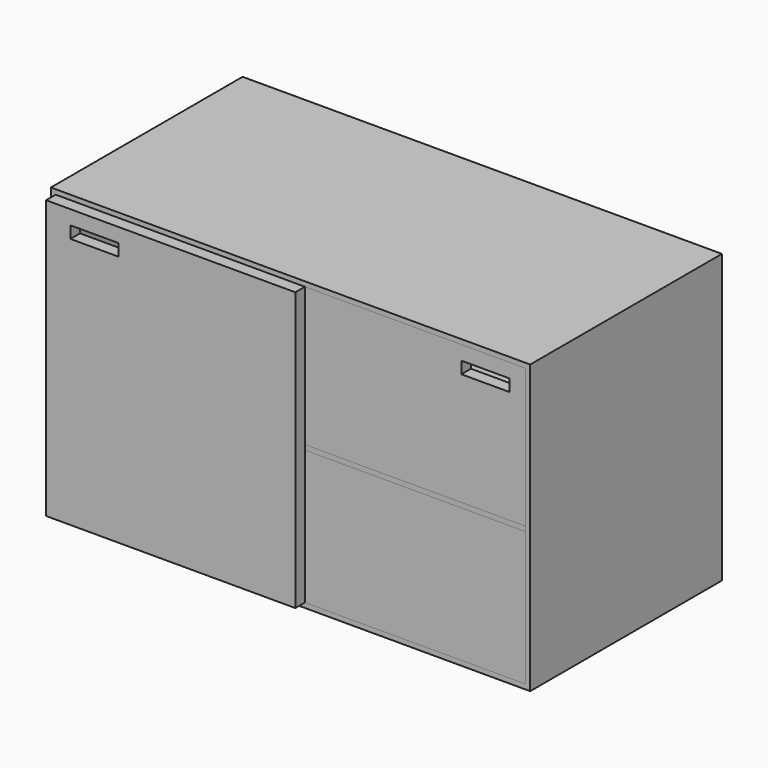
from build123d import *

# Parameters (mm, degrees)
F0_W          = 1000
F0_H          = 600
F1_DEPTH      = 500
F2_T          = -10
F3_W          = 460
F3_H          = 580
F3_W_2        = 60
F4_DEPTH      = 25
F5_DEPTH      = 25
F6_W          = 100
F6_H          = 25
F7_DEPTH      = 525.001
F7_DEPTH_BACK = 1899
F8_W          = 980
F8_H          = 10
F9_DEPTH      = 490
F10_W         = 10
F10_H         = 580
F11_DEPTH     = 490


# Not quite as in the source:
# - an extrude ends at something that could not be found from the text; its depth is read off the source's solid


with BuildPart() as f1:
    # F0 (on Front) → F1 (new body)
    with BuildSketch(Plane.XZ):
        with Locations((500, 300)):
            Rectangle(F0_W, F0_H)
    extrude(amount=F1_DEPTH)

    # F2
    f2_openings = [f1.faces().sort_by_distance(p)[0] for p in [
        (500, -500, 300),
    ]]
    offset(amount=F2_T, openings=f2_openings)


with BuildPart() as f4:
    # F3 (on face) → F4 (new body)
    with BuildSketch(Plane.XZ.offset(500)):
        with Locations((240, 300)):
            Rectangle(F3_W, F3_H)
        with Locations((500, 300)):
            Rectangle(F3_W_2, F3_H)
    extrude(amount=F4_DEPTH)


with BuildPart() as f5:
    # F3 (on face) → F5 (new body)
    with BuildSketch(Plane.XZ.offset(500)):
        with Locations((760, 300)):
            Rectangle(F3_W, F3_H)
        with Locations((500, 300)):
            Rectangle(F3_W_2, F3_H)
    extrude(amount=-F5_DEPTH)


with BuildPart() as f7_tool:
    # F6 (on face) → F7 (new body, two sides)
    with BuildSketch(Plane.XZ.offset(525)) as f7_sk:
        with Locations((110.8831882477, 547.9354381561)):
            Rectangle(F6_W, F6_H)
        with Locations((906.3955426216, 547.9354381561)):
            Rectangle(F6_W, F6_H)
    extrude(amount=-F7_DEPTH)
    extrude(f7_sk.sketch, amount=F7_DEPTH_BACK)


with BuildPart() as f4_1:
    add(f4.part)

    # F7: cut by f7_tool
    add(f7_tool.part, mode=Mode.SUBTRACT)


with BuildPart() as f5_1:
    add(f5.part)

    # F7: cut by f7_tool
    add(f7_tool.part, mode=Mode.SUBTRACT)


with BuildPart() as f9:
    # F8 (on face) → F9 (new body, through all)
    with BuildSketch(Plane.XZ.offset(10)):
        with Locations((500, 295)):
            Rectangle(F8_W, F8_H)
    extrude(amount=F9_DEPTH)


with BuildPart() as f11:
    # F10 (on face) → F11 (new body, through all)
    with BuildSketch(Plane.XZ.offset(10)):
        with Locations((495, 300)):
            Rectangle(F10_W, F10_H)
    extrude(amount=F11_DEPTH)


solid = Compound([f1.part, f4_1.part, f5_1.part, f9.part, f11.part])
